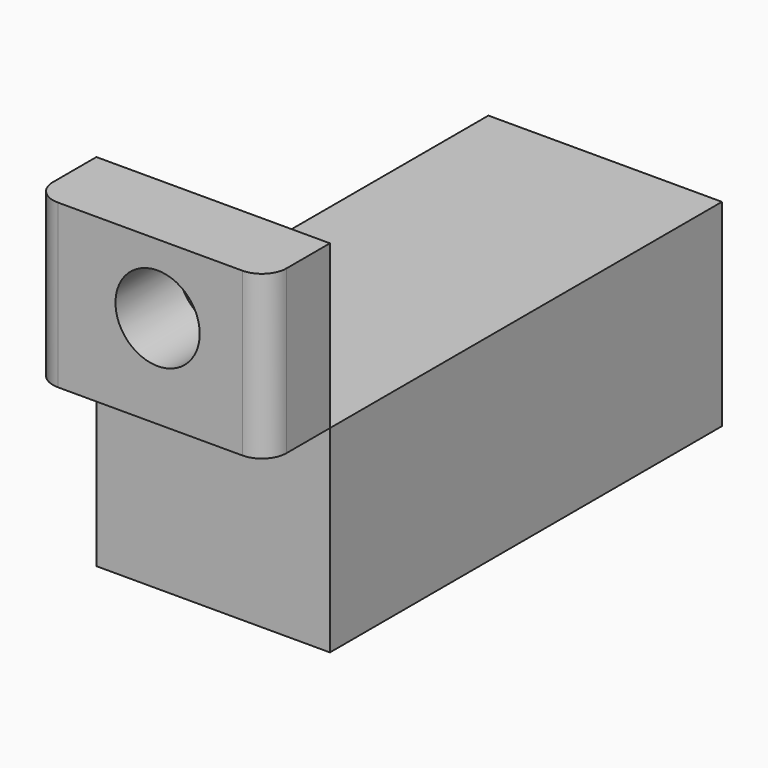
from build123d import *

# Parameters (mm, degrees)
F0_W     = 60.5307035148
F0_H     = 51.193524152
F1_DEPTH = 127
F3_DEPTH = 42.164
F4_R     = 10.922
F5_DEPTH = 25.4


# Not quite as in the source:
# - the program builds the solid bodies; features that only make, move or delete a surface that nothing else refers to are left out


with BuildPart() as f1:
    # F0 (on Front) → F1 (new body)
    with BuildSketch(Plane.XZ):
        Rectangle(F0_W, F0_H)
    extrude(amount=F1_DEPTH)


with BuildPart() as f3:
    # F2 (on face) → F3 (new body)
    with BuildSketch(Plane.XY.offset(25.596762076)):
        with BuildLine():
            Line((30.2653517574, -127), (-30.2653517574, -127))
            Line((-30.2653517574, -127), (-30.2653517574, -141.0862502229))
            ThreePointArc((-30.2653517574, -141.0862502229), (-28.4054798179, -145.5763782835), (-23.9153517574, -147.4362502229))
            Line((-23.9153517574, -147.4362502229), (23.9153517574, -147.4362502229))
            ThreePointArc((23.9153517574, -147.4362502229), (28.4054798179, -145.5763782835), (30.2653517574, -141.0862502229))
            Line((30.2653517574, -141.0862502229), (30.2653517574, -127))
        make_face()
    extrude(amount=F3_DEPTH)

    # F4 (on face) → F5 (cut)
    with BuildSketch(Plane.XZ.offset(147.4362502229)):
        with Locations((1.9451410044, 49.7585572302)):
            Circle(F4_R)
    extrude(amount=-F5_DEPTH, mode=Mode.SUBTRACT)


solid = Compound([f1.part, f3.part])
